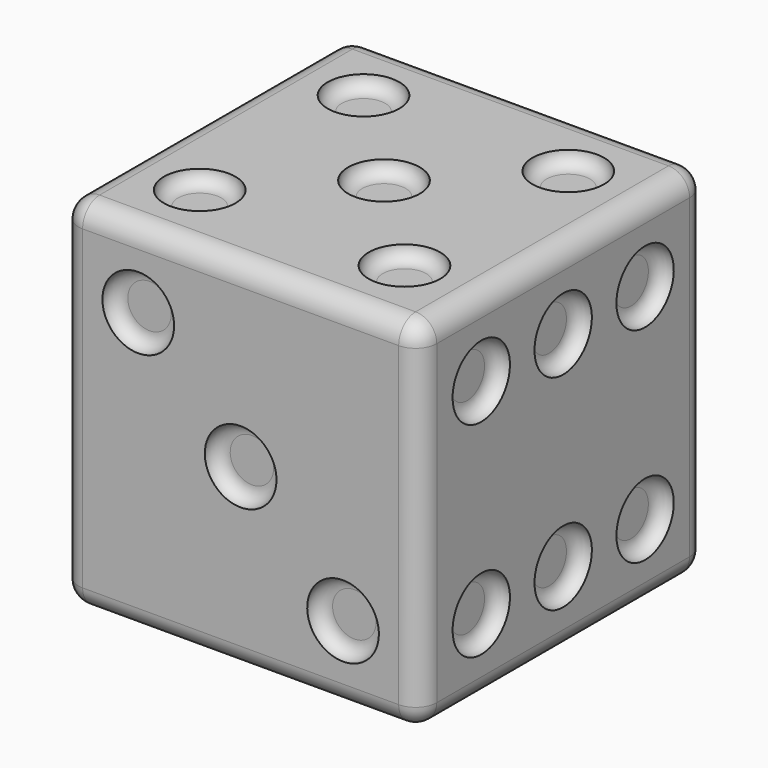
from build123d import *

# Parameters (mm, degrees)
F2_W          = 25.4
F2_H          = 25.4
F3_DEPTH      = 25.4
F4_R          = 2.54
F10_DEPTH     = 1
F11_R         = 0.99999
F5_R          = 2.54
F12_DEPTH     = 1
F13_R         = 0.99999
F9_R          = 2.54
F14_DEPTH     = 1
F15_R         = 0.99999
F6_R          = 2.54
F16_DEPTH     = 1
F17_R         = 0.99999
F7_R          = 2.54
F18_DEPTH     = 1
F19_R         = 0.99999
F8_R          = 2.54
F20_DEPTH     = 1
F21_R         = 0.99999
F22_R         = 1.5
F23_R         = 1.5
F24_T1_DEPTH  = 22.4
F24_S5_W      = 1.5
F24_S5_H      = 1.5
F24_T6_DEPTH  = 1.5
F24_S11_W     = 1.5
F24_S11_H     = 1.5
F24_T12_DEPTH = 1.5
F24_S17_W     = 1.5
F24_S17_H     = 1.5
F24_T18_DEPTH = 1.5
F24_S23_W     = 1.5
F24_S23_H     = 1.5
F24_T24_DEPTH = 1.5
F24_S29_W     = 1.5
F24_S29_H     = 1.5
F24_T30_DEPTH = 1.5
F24_S35_W     = 1.5
F24_S35_H     = 1.5
F24_T36_DEPTH = 1.5
F24_S41_W     = 1.5
F24_S41_H     = 1.5
F24_T42_DEPTH = 1.5
F24_S47_W     = 1.5
F24_S47_H     = 1.5
F24_T48_DEPTH = 1.5
F27_ANGLE     = 90


# Not quite as in the source:
# - a fillet or chamfer that OpenCascade refuses, or shapes differently, is made with other operations: its cross-section is extruded or revolved along the edge and cut away or added
# - a fillet or chamfer is up to 0.001 mm smaller than in the source, because OpenCascade refuses the exact size


with BuildPart() as f3:
    # F2 (on Top) → F3 (new body)
    with BuildSketch(Plane.XY):
        Rectangle(F2_W, F2_H)
    extrude(amount=F3_DEPTH)

    # F4 (on face) → F10 (cut)
    with BuildSketch(Plane(origin=(0, 0, 0), x_dir=(1, 0, 0), z_dir=(0, 0, -1))):
        with Locations((7.2571428571, 7.2571428571)):
            Circle(F4_R)
        with Locations((7.2571428571, 0)):
            Circle(F4_R)
        with Locations((7.2571428571, -7.2571428571)):
            Circle(F4_R)
        with Locations((-7.2571428571, -7.2571428571)):
            Circle(F4_R)
        with Locations((-7.2571428571, 0)):
            Circle(F4_R)
        with Locations((-7.2571428571, 7.2571428571)):
            Circle(F4_R)
    extrude(amount=-F10_DEPTH, mode=Mode.SUBTRACT)

    # F11 (radius 1 in the source; OpenCascade refuses exactly that, so slightly less here)
    f11_edges = [f3.edges().sort_by_distance(p)[0] for p in [
        (4.717143, 7.257143, 1),
        (-9.797143, 7.257143, 1),
        (4.717143, 0, 1),
        (4.717143, -7.257143, 1),
        (-9.797143, 0, 1),
        (-9.797143, -7.257143, 1),
    ]]
    fillet(f11_edges, radius=F11_R)

    # F5 (on face) → F12 (cut)
    with BuildSketch(Plane.XY.offset(25.4)):
        Circle(F5_R)
    extrude(amount=-F12_DEPTH, mode=Mode.SUBTRACT)

    # F13 (radius 1 in the source; OpenCascade refuses exactly that, so slightly less here)
    f13_edges = [f3.edges().sort_by_distance(p)[0] for p in [
        (-2.54, 0, 24.4),
    ]]
    fillet(f13_edges, radius=F13_R)

    # F9 (on face) → F14 (cut)
    with BuildSketch(Plane.XZ.offset(12.7)):
        with Locations((7.2571428571, 19.9571428571)):
            Circle(F9_R)
        with Locations((0, 12.7)):
            Circle(F9_R)
        with Locations((-7.2571428571, 5.4428571429)):
            Circle(F9_R)
    extrude(amount=-F14_DEPTH, mode=Mode.SUBTRACT)

    # F15 (radius 1 in the source; OpenCascade refuses exactly that, so slightly less here)
    f15_edges = [f3.edges().sort_by_distance(p)[0] for p in [
        (4.717143, -11.7, 19.957143),
        (-2.54, -11.7, 12.7),
        (-9.797143, -11.7, 5.442857),
    ]]
    fillet(f15_edges, radius=F15_R)

    # F6 (on face) → F16 (cut)
    with BuildSketch(Plane.YZ.offset(12.7)):
        with Locations((-7.2571428571, 19.9571428571)):
            Circle(F6_R)
        with Locations((-7.2571428571, 5.4428571429)):
            Circle(F6_R)
        with Locations((7.2571428571, 19.9571428571)):
            Circle(F6_R)
        with Locations((0, 12.7)):
            Circle(F6_R)
        with Locations((7.2571428571, 5.4428571429)):
            Circle(F6_R)
    extrude(amount=-F16_DEPTH, mode=Mode.SUBTRACT)

    # F17 (radius 1 in the source; OpenCascade refuses exactly that, so slightly less here)
    f17_edges = [f3.edges().sort_by_distance(p)[0] for p in [
        (11.7, -9.797143, 5.442857),
        (11.7, -9.797143, 19.957143),
        (11.7, -2.54, 12.7),
        (11.7, 4.717143, 5.442857),
        (11.7, 4.717143, 19.957143),
    ]]
    fillet(f17_edges, radius=F17_R)

    # F7 (on face) → F18 (cut)
    with BuildSketch(Plane(origin=(0, 12.7, 0), x_dir=(-1, 0, 0), z_dir=(0, 1, 0))):
        with Locations((-7.2571428571, 19.9571428571)):
            Circle(F7_R)
        with Locations((-7.2571428571, 5.4428571429)):
            Circle(F7_R)
        with Locations((7.2571428571, 19.9571428571)):
            Circle(F7_R)
        with Locations((7.2571428571, 5.4428571429)):
            Circle(F7_R)
    extrude(amount=-F18_DEPTH, mode=Mode.SUBTRACT)

    # F19 (radius 1 in the source; OpenCascade refuses exactly that, so slightly less here)
    f19_edges = [f3.edges().sort_by_distance(p)[0] for p in [
        (9.797143, 11.7, 5.442857),
        (9.797143, 11.7, 19.957143),
        (-4.717143, 11.7, 19.957143),
        (-4.717143, 11.7, 5.442857),
    ]]
    fillet(f19_edges, radius=F19_R)

    # F8 (on face) → F20 (cut)
    with BuildSketch(Plane(origin=(-12.7, 0, 0), x_dir=(0, -1, 0), z_dir=(-1, 0, 0))):
        with Locations((7.2571428571, 5.4428571429)):
            Circle(F8_R)
        with Locations((-7.2571428571, 19.9571428571)):
            Circle(F8_R)
    extrude(amount=-F20_DEPTH, mode=Mode.SUBTRACT)

    # F21 (radius 1 in the source; OpenCascade refuses exactly that, so slightly less here)
    f21_edges = [f3.edges().sort_by_distance(p)[0] for p in [
        (-11.7, 9.797143, 19.957143),
        (-11.7, -4.717143, 5.442857),
    ]]
    fillet(f21_edges, radius=F21_R)

    # F22
    f22_edges = [f3.edges().sort_by_distance(p)[0] for p in [
        (0, -12.7, 25.4),
        (12.7, 0, 25.4),
        (0, 12.7, 25.4),
        (-12.7, 0, 25.4),
    ]]
    fillet(f22_edges, radius=F22_R)

    # F23
    f23_edges = [f3.edges().sort_by_distance(p)[0] for p in [
        (0, -12.7, 0),
        (12.7, 0, 0),
        (0, 12.7, 0),
        (-12.7, 0, 0),
    ]]
    fillet(f23_edges, radius=F23_R)

    # F24: fillet of radius 1.5 on 4 edges, made by hand

    # F24_s2 → F24_t1 (cut)
    with BuildSketch(Plane.XY.offset(1.5)):
        with BuildLine():
            ThreePointArc((-12.7, -11.2), (-12.2606601718, -12.2606601718), (-11.2, -12.7))
            Line((-11.2, -12.7), (-12.7, -12.7))
            Line((-12.7, -12.7), (-12.7, -11.2))
        make_face()
        with BuildLine():
            ThreePointArc((11.2, -12.7), (12.2606601718, -12.2606601718), (12.7, -11.2))
            Line((12.7, -11.2), (12.7, -12.7))
            Line((12.7, -12.7), (11.2, -12.7))
        make_face()
        with BuildLine():
            ThreePointArc((11.2, 12.7), (12.2606601718, 12.2606601718), (12.7, 11.2))
            Line((12.7, 11.2), (12.7, 12.7))
            Line((12.7, 12.7), (11.2, 12.7))
        make_face()
        with BuildLine():
            ThreePointArc((-12.7, 11.2), (-12.2606601718, 12.2606601718), (-11.2, 12.7))
            Line((-11.2, 12.7), (-12.7, 12.7))
            Line((-12.7, 12.7), (-12.7, 11.2))
        make_face()
    extrude(amount=F24_T1_DEPTH, mode=Mode.SUBTRACT)


with BuildPart() as f24_tool4:
    # F24_s5 → F24_t6 (new body)
    with BuildSketch(Plane.YZ.offset(-11.2)):
        with Locations((11.95, 0.75)):
            Rectangle(F24_S5_W, F24_S5_H)
    extrude(amount=-F24_T6_DEPTH)

    # F24_s7 → F24_t8 (revolve, cut)
    with BuildSketch(Plane(origin=(-11.2, 11.2, 1.5), x_dir=(0, -0.7071067812, 0.7071067812), z_dir=(0, -0.7071067812, -0.7071067812))):
        with BuildLine():
            ThreePointArc((0, -1.5), (1.5, 0), (0, 1.5))
            Line((0, 1.5), (0, -1.5))
        make_face()
    revolve(axis=Axis((-11.2, 11.2, 1.5), (-1, 0, 0)), mode=Mode.SUBTRACT)


with BuildPart() as f3_1:
    add(f3.part)

    # F24_t3: cut F24_tool4
    add(f24_tool4.part, mode=Mode.SUBTRACT)


with BuildPart() as f24_tool10:
    # F24_s11 → F24_t12 (new body)
    with BuildSketch(Plane.YZ.offset(-11.2)):
        with Locations((11.95, 24.65)):
            Rectangle(F24_S11_W, F24_S11_H)
    extrude(amount=-F24_T12_DEPTH)

    # F24_s13 → F24_t14 (revolve, cut)
    with BuildSketch(Plane(origin=(-11.2, 11.2, 23.9), x_dir=(0, -0.7071067812, -0.7071067812), z_dir=(0, 0.7071067812, -0.7071067812))):
        with BuildLine():
            ThreePointArc((0, -1.5), (1.5, 0), (0, 1.5))
            Line((0, 1.5), (0, -1.5))
        make_face()
    revolve(axis=Axis((-11.2, 11.2, 23.9), (-1, 0, 0)), mode=Mode.SUBTRACT)


with BuildPart() as f3_2:
    add(f3_1.part)

    # F24_t9: cut F24_tool10
    add(f24_tool10.part, mode=Mode.SUBTRACT)


with BuildPart() as f24_tool16:
    # F24_s17 → F24_t18 (new body)
    with BuildSketch(Plane.XZ.offset(-11.2)):
        with Locations((11.95, 0.75)):
            Rectangle(F24_S17_W, F24_S17_H)
    extrude(amount=-F24_T18_DEPTH)

    # F24_s19 → F24_t20 (revolve, cut)
    with BuildSketch(Plane(origin=(11.2, 11.2, 1.5), x_dir=(-0.7071067812, 0, 0.7071067812), z_dir=(-0.7071067812, 0, -0.7071067812))):
        with BuildLine():
            ThreePointArc((0, -1.5), (1.5, 0), (0, 1.5))
            Line((0, 1.5), (0, -1.5))
        make_face()
    revolve(axis=Axis((11.2, 11.2, 1.5), (0, 1, 0)), mode=Mode.SUBTRACT)


with BuildPart() as f3_3:
    add(f3_2.part)

    # F24_t15: cut F24_tool16
    add(f24_tool16.part, mode=Mode.SUBTRACT)


with BuildPart() as f24_tool22:
    # F24_s23 → F24_t24 (new body)
    with BuildSketch(Plane.XZ.offset(-11.2)):
        with Locations((11.95, 24.65)):
            Rectangle(F24_S23_W, F24_S23_H)
    extrude(amount=-F24_T24_DEPTH)

    # F24_s25 → F24_t26 (revolve, cut)
    with BuildSketch(Plane(origin=(11.2, 11.2, 23.9), x_dir=(-0.7071067812, 0, -0.7071067812), z_dir=(0.7071067812, 0, -0.7071067812))):
        with BuildLine():
            ThreePointArc((0, -1.5), (1.5, 0), (0, 1.5))
            Line((0, 1.5), (0, -1.5))
        make_face()
    revolve(axis=Axis((11.2, 11.2, 23.9), (0, 1, 0)), mode=Mode.SUBTRACT)


with BuildPart() as f3_4:
    add(f3_3.part)

    # F24_t21: cut F24_tool22
    add(f24_tool22.part, mode=Mode.SUBTRACT)


with BuildPart() as f24_tool28:
    # F24_s29 → F24_t30 (new body)
    with BuildSketch(Plane.XZ.offset(11.2)):
        with Locations((11.95, 0.75)):
            Rectangle(F24_S29_W, F24_S29_H)
    extrude(amount=F24_T30_DEPTH)

    # F24_s31 → F24_t32 (revolve, cut)
    with BuildSketch(Plane(origin=(11.2, -11.2, 1.5), x_dir=(-0.7071067812, 0, 0.7071067812), z_dir=(0.7071067812, 0, 0.7071067812))):
        with BuildLine():
            ThreePointArc((0, -1.5), (1.5, 0), (0, 1.5))
            Line((0, 1.5), (0, -1.5))
        make_face()
    revolve(axis=Axis((11.2, -11.2, 1.5), (0, -1, 0)), mode=Mode.SUBTRACT)


with BuildPart() as f3_5:
    add(f3_4.part)

    # F24_t27: cut F24_tool28
    add(f24_tool28.part, mode=Mode.SUBTRACT)


with BuildPart() as f24_tool34:
    # F24_s35 → F24_t36 (new body)
    with BuildSketch(Plane.XZ.offset(11.2)):
        with Locations((11.95, 24.65)):
            Rectangle(F24_S35_W, F24_S35_H)
    extrude(amount=F24_T36_DEPTH)

    # F24_s37 → F24_t38 (revolve, cut)
    with BuildSketch(Plane(origin=(11.2, -11.2, 23.9), x_dir=(-0.7071067812, 0, -0.7071067812), z_dir=(-0.7071067812, 0, 0.7071067812))):
        with BuildLine():
            ThreePointArc((0, -1.5), (1.5, 0), (0, 1.5))
            Line((0, 1.5), (0, -1.5))
        make_face()
    revolve(axis=Axis((11.2, -11.2, 23.9), (0, -1, 0)), mode=Mode.SUBTRACT)


with BuildPart() as f3_6:
    add(f3_5.part)

    # F24_t33: cut F24_tool34
    add(f24_tool34.part, mode=Mode.SUBTRACT)


with BuildPart() as f24_tool40:
    # F24_s41 → F24_t42 (new body)
    with BuildSketch(Plane.YZ.offset(-11.2)):
        with Locations((-11.95, 0.75)):
            Rectangle(F24_S41_W, F24_S41_H)
    extrude(amount=-F24_T42_DEPTH)

    # F24_s43 → F24_t44 (revolve, cut)
    with BuildSketch(Plane(origin=(-11.2, -11.2, 1.5), x_dir=(0, 0.7071067812, 0.7071067812), z_dir=(0, -0.7071067812, 0.7071067812))):
        with BuildLine():
            ThreePointArc((0, -1.5), (1.5, 0), (0, 1.5))
            Line((0, 1.5), (0, -1.5))
        make_face()
    revolve(axis=Axis((-11.2, -11.2, 1.5), (-1, 0, 0)), mode=Mode.SUBTRACT)


with BuildPart() as f3_7:
    add(f3_6.part)

    # F24_t39: cut F24_tool40
    add(f24_tool40.part, mode=Mode.SUBTRACT)


with BuildPart() as f24_tool46:
    # F24_s47 → F24_t48 (new body)
    with BuildSketch(Plane.YZ.offset(-11.2)):
        with Locations((-11.95, 24.65)):
            Rectangle(F24_S47_W, F24_S47_H)
    extrude(amount=-F24_T48_DEPTH)

    # F24_s49 → F24_t50 (revolve, cut)
    with BuildSketch(Plane(origin=(-11.2, -11.2, 23.9), x_dir=(0, 0.7071067812, -0.7071067812), z_dir=(0, 0.7071067812, 0.7071067812))):
        with BuildLine():
            ThreePointArc((0, -1.5), (1.5, 0), (0, 1.5))
            Line((0, 1.5), (0, -1.5))
        make_face()
    revolve(axis=Axis((-11.2, -11.2, 23.9), (-1, 0, 0)), mode=Mode.SUBTRACT)


with BuildPart() as f3_8:
    add(f3_7.part)

    # F24_t45: cut F24_tool46
    add(f24_tool46.part, mode=Mode.SUBTRACT)


with BuildPart() as f3_9:
    # F27: moved
    add(f3_8.part.rotate(Axis((0, 0, 12.7), (0, -1, 0)), F27_ANGLE))


solid = f3_9.part
